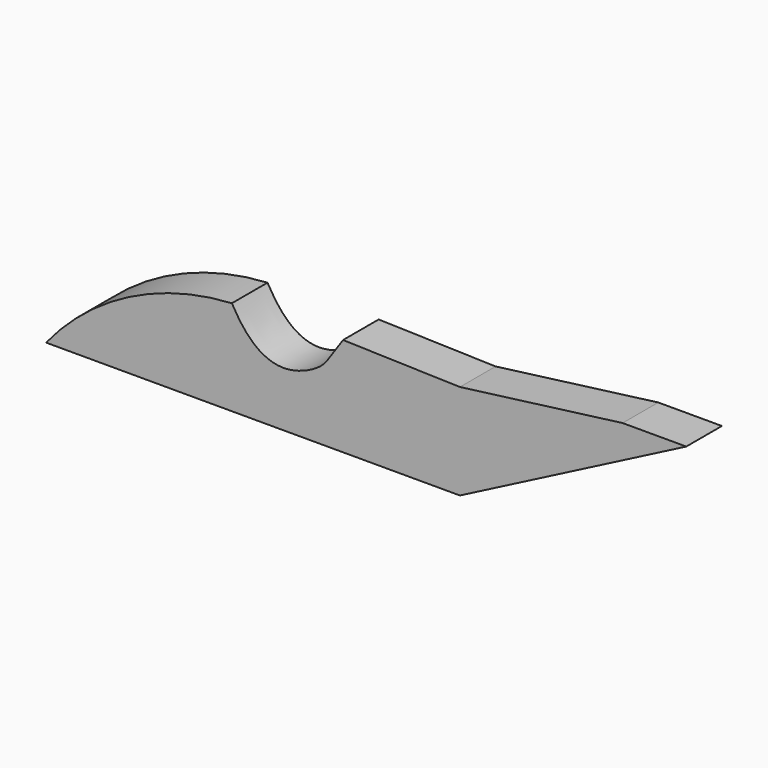
from build123d import *

# Parameters (mm, degrees)
F1_DEPTH    = 17.78
F2_T1_DEPTH = 417.7319430625


# Not quite as in the source:
# - a fillet or chamfer that OpenCascade refuses, or shapes differently, is made with other operations: its cross-section is extruded or revolved along the edge and cut away or added


with BuildPart() as f1:
    # F0 (on Front) → F1 (new body)
    with BuildSketch(Plane.XZ):
        with BuildLine():
            Line((-162.0961189375, -1.346105228), (-162.0961189375, -39.446105228))
            Line((-162.0961189375, -39.446105228), (3.0038810625, -39.446105228))
            Line((3.0038810625, -39.446105228), (93.3108132751, 7.1072834172))
            Line((93.3108132751, 7.1072834172), (67.9108132751, 7.1072834172))
            Line((67.9108132751, 7.1072834172), (3.0038810625, -1.346105228))
            Line((3.0038810625, -1.346105228), (-43.6204448342, 0))
            add(Edge.make_bspline(
                [(-88.0704448342, -1.346105228), (-85.1866431635, -6.6508062653), (-78.8098016913, -15.013308036), (-66.0558603131, -19.2294666036), (-50.4728148138, -12.3489722112), (-48.5910698771, -6.9073382765), (-43.6204448342, 0)],
                knots=[0, 0, 0, 0, 0.2654455487, 0.4966311992, 0.7427406625, 1, 1, 1, 1], degree=3))
            Line((-88.0704448342, -1.346105228), (-162.0961189375, -1.346105228))
        make_face()
    extrude(amount=F1_DEPTH)

    # F2: fillet of radius 103.0193211336 on 1 edges, made by hand

    # F2_s2 → F2_t1 (cut)
    with BuildSketch(Plane.XZ.offset(-199.9759715313)):
        with BuildLine():
            ThreePointArc((-82.105730325, -1.346105228), (-126.4060471139, -11.3575640099), (-162.0961189375, -39.446105228))
            Line((-162.0961189375, -39.446105228), (-162.0961189375, -1.346105228))
            Line((-162.0961189375, -1.346105228), (-82.105730325, -1.346105228))
        make_face()
    extrude(amount=F2_T1_DEPTH, mode=Mode.SUBTRACT)


solid = f1.part
